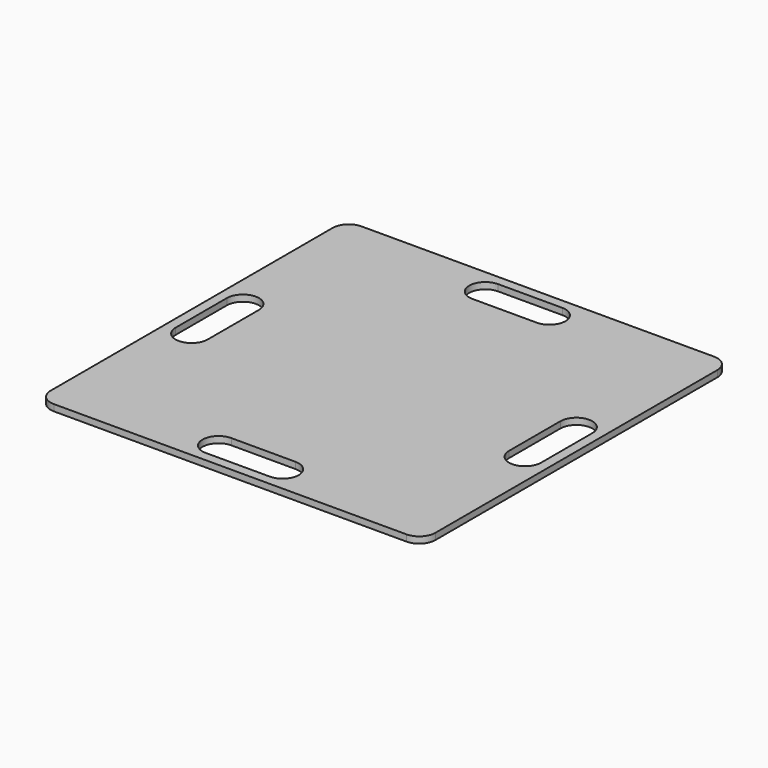
from build123d import *

# Parameters (mm, degrees)
F0_W            = 600
F0_H            = 600
F1_DEPTH        = 10
F3_DEPTH        = 10.001
F3_COPIES_COUNT = 4
F5_R            = 25


# Not quite as in the source:
# - a pattern or mirror of a feature is missing from the dataset's text; its kind, count and spacing are read off the source's solid


with BuildPart() as f1:
    # F0 (on Top) → F1 (new body)
    with BuildSketch(Plane.XY):
        Rectangle(F0_W, F0_H)
    extrude(amount=F1_DEPTH)

    # F2 (on Top) → F3 (cut, through all)
    with BuildSketch(Plane.XY):
        with BuildLine():
            Line((-50, 235), (50, 235))
            ThreePointArc((50, 235), (75, 260), (50, 285))
            Line((50, 285), (-50, 285))
            ThreePointArc((-50, 285), (-75, 260), (-50, 235))
        make_face()
    f3 = extrude(amount=F3_DEPTH, mode=Mode.SUBTRACT)

    # F3_copies: F3 ×4 about axis
    f3_copies_axis = Axis((0, 0, 0), (0, 0, 1))
    for i in range(1, F3_COPIES_COUNT):
        add(f3.rotate(f3_copies_axis, i * 360 / F3_COPIES_COUNT), mode=Mode.SUBTRACT)

    # F5
    f5_edges = [f1.edges().sort_by_distance(p)[0] for p in [
        (-300, -300, 5),
        (-300, 300, 5),
        (300, 300, 5),
        (300, -300, 5),
    ]]
    fillet(f5_edges, radius=F5_R)


solid = f1.part
